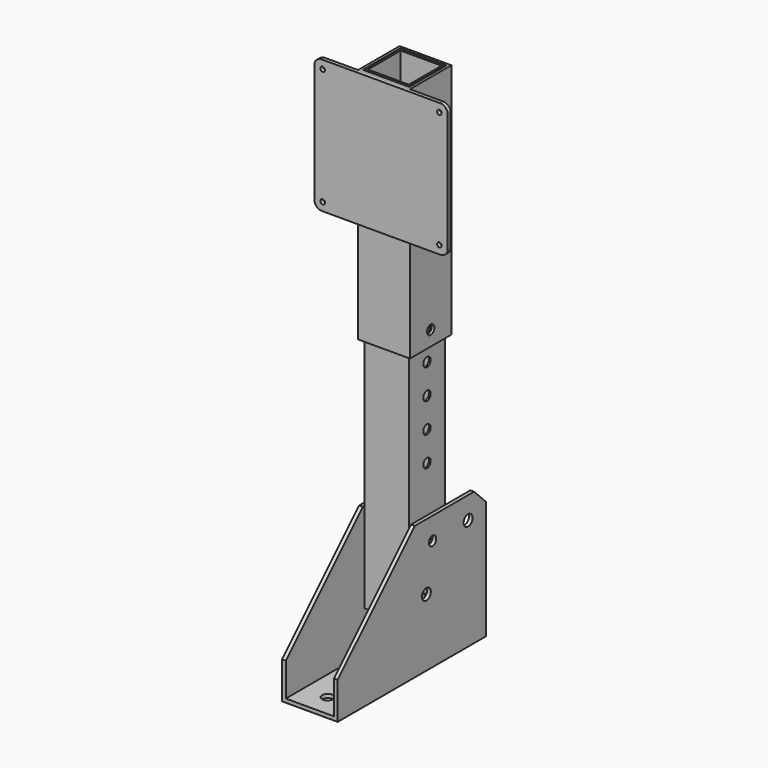
from build123d import *

# Parameters (mm, degrees)
F0_W      = 114.3
F0_H      = 114.3
F0_R      = 2
F1_DEPTH  = 3.175
F2_R      = 6.35
F3_W      = 44.45
F3_H      = 44.45
F3_W_2    = 39.878
F3_H_2    = 39.878
F4_DEPTH  = 203.2
F6_R      = 4.7625
F6_R_2    = 3.96875
F7_DEPTH  = 23.8125
F8_T      = -3.175
F9_W      = 38.1
F9_H      = 406.4
F9_R      = 3.96875
F10_DEPTH = 19.05
F11_T     = -1.524
F12_R     = 3.96875
F13_DEPTH = 50.8
F14_R     = 3.96875
F15_DEPTH = 50.8
F16_R     = 4.7625
F17_DEPTH = 25.4
F18_R     = 4.7625
F19_DEPTH = 25.4
F20_SIZE  = 12.7


with BuildPart() as f1:
    # F0 (on Front) → F1 (new body)
    with BuildSketch(Plane.XZ):
        Rectangle(F0_W, F0_H)
        with Locations((-50, -50)):
            Circle(F0_R, mode=Mode.SUBTRACT)
        with Locations((50, -50)):
            Circle(F0_R, mode=Mode.SUBTRACT)
        with Locations((-50, 50)):
            Circle(F0_R, mode=Mode.SUBTRACT)
        with Locations((50, 50)):
            Circle(F0_R, mode=Mode.SUBTRACT)
    extrude(amount=F1_DEPTH)

    # F2
    f2_edges = [f1.edges().sort_by_distance(p)[0] for p in [
        (-57.15, -1.5875, 57.15),
        (57.15, -1.5875, 57.15),
        (-57.15, -1.5875, -57.15),
        (57.15, -1.5875, -57.15),
    ]]
    fillet(f2_edges, radius=F2_R)


with BuildPart() as f4:
    # F3 (on face) → F4 (new body)
    with BuildSketch(Plane.XY.offset(57.15)):
        with Locations((0, 22.225)):
            Rectangle(F3_W, F3_H)
        with Locations((0, 22.225)):
            Rectangle(F3_W_2, F3_H_2, mode=Mode.SUBTRACT)
    extrude(amount=-F4_DEPTH)


with BuildPart() as f7:
    # F6 (on Right) → F7 (new body, symmetric)
    with BuildSketch(Plane.YZ):
        Polygon((-79.375, -387.35), (3.175, -387.35), (79.375, -387.35), (79.375, -273.05), (3.175, -273.05), (-79.375, -355.6), align=None)
        with Locations((15.6090044309, -329.6211753898)):
            Circle(F6_R, mode=Mode.SUBTRACT)
        with Locations((22.225, -292.1)):
            Circle(F6_R_2, mode=Mode.SUBTRACT)
        with Locations((60.325, -292.1)):
            Circle(F6_R, mode=Mode.SUBTRACT)
    extrude(amount=F7_DEPTH, both=True)

    # F8
    f8_openings = [f7.faces().sort_by_distance(p)[0] for p in [
        (0, 79.375, -330.2),
        (0, 41.275, -273.05),
        (0, 10.846504, -329.621175),
        (0, 18.25625, -292.1),
        (0, 55.5625, -292.1),
        (0, -79.375, -371.475),
        (0, -38.1, -314.325),
    ]]
    offset(amount=F8_T, openings=f8_openings)

    # F16 (on face) → F17 (cut)
    with BuildSketch(Plane(origin=(0, 0, -387.35), x_dir=(1, 0, 0), z_dir=(0, 0, -1))):
        with Locations((0, -15.875)):
            Circle(F16_R)
        with Locations((0, -66.675)):
            Circle(F16_R)
    extrude(amount=-F17_DEPTH, mode=Mode.SUBTRACT)

    # F18 (on face) → F19 (cut)
    with BuildSketch(Plane.XY.offset(-384.175)):
        with Locations((0, -60.325)):
            Circle(F18_R)
    extrude(amount=-F19_DEPTH, mode=Mode.SUBTRACT)

    # F20
    f20_edges = [f7.edges().sort_by_distance(p)[0] for p in [
        (-22.225, 79.375, -273.05),
        (22.225, 79.375, -273.05),
    ]]
    chamfer(f20_edges, length=F20_SIZE)


with BuildPart() as f10:
    # F9 (on Right) → F10 (new body, symmetric)
    with BuildSketch(Plane.YZ):
        with Locations((22.225, -146.05)):
            Rectangle(F9_W, F9_H)
        with Locations((22.310306693, -330.1999044981)):
            Circle(F9_R, mode=Mode.SUBTRACT)
        with Locations((22.225, -292.1)):
            Circle(F9_R, mode=Mode.SUBTRACT)
    extrude(amount=F10_DEPTH, both=True)

    # F11
    f11_openings = [f10.faces().sort_by_distance(p)[0] for p in [
        (0, 22.225, 57.15),
        (0, 18.25625, -292.1),
        (0, 22.225, -349.25),
        (0, 18.341557, -330.199904),
    ]]
    offset(amount=F11_T, openings=f11_openings)


with BuildPart() as f13_tool:
    # F12 (on Right) → F13 (new body, symmetric)
    with BuildSketch(Plane.YZ):
        with Locations((22.225, -133.35)):
            Circle(F12_R)
    extrude(amount=F13_DEPTH, both=True)


with BuildPart() as f4_1:
    add(f4.part)

    # F13: cut by f13_tool
    add(f13_tool.part, mode=Mode.SUBTRACT)


with BuildPart() as f10_1:
    add(f10.part)

    # F13: cut by f13_tool
    add(f13_tool.part, mode=Mode.SUBTRACT)

    # F14 (on face) → F15 (cut, symmetric)
    with BuildSketch(Plane.YZ.offset(19.05)):
        with Locations((22.225, -6.35)):
            Circle(F14_R)
        with Locations((22.225, -31.75)):
            Circle(F14_R)
        with Locations((22.225, -57.15)):
            Circle(F14_R)
        with Locations((22.225, -82.55)):
            Circle(F14_R)
        with Locations((22.225, -107.95)):
            Circle(F14_R)
        with Locations((22.225, -133.35)):
            Circle(F14_R)
        with Locations((22.225, -158.75)):
            Circle(F14_R)
        with Locations((22.225, -184.15)):
            Circle(F14_R)
        with Locations((22.225, -209.55)):
            Circle(F14_R)
        with Locations((22.225, -234.95)):
            Circle(F14_R)
    extrude(amount=F15_DEPTH, both=True, mode=Mode.SUBTRACT)


solid = Compound([f1.part, f7.part, f4_1.part, f10_1.part])
